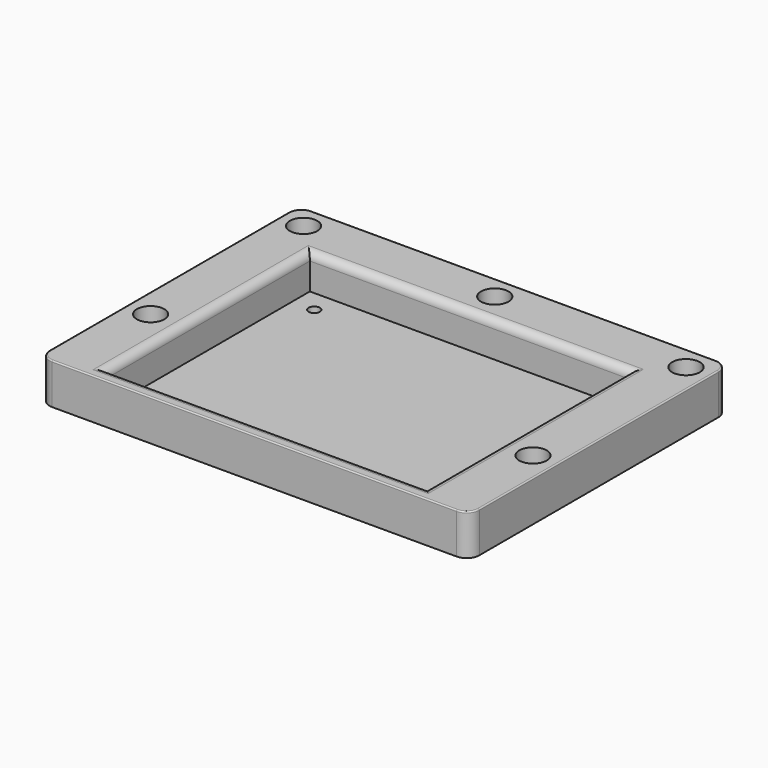
from build123d import *

# Parameters (mm, degrees)
F0_W          = 128.778
F0_H          = 102.108
F1_DEPTH      = 2.54
F2_W          = 173.228
F2_H          = 130.683
F2_W_2        = 128.778
F2_H_2        = 102.108
F3_DEPTH      = 16.51
F4_R          = 3.175
F5_R          = 5.55625
F6_DEPTH      = 16.511
F7_R          = 2.2479
F8_DEPTH      = 2.541
F9_R          = 0.508
F10_T1_DEPTH  = 29.21
F10_T4_ANGLE  = 90
F10_T6_ANGLE  = 90
F10_T8_ANGLE  = 90
F10_T10_ANGLE = 90


# Not quite as in the source:
# - a fillet or chamfer that OpenCascade refuses, or shapes differently, is made with other operations: its cross-section is extruded or revolved along the edge and cut away or added


with BuildPart() as f1:
    # F0 (on Top) → F1 (new body)
    with BuildSketch(Plane.XY):
        Rectangle(F0_W, F0_H)
    extrude(amount=F1_DEPTH)

    # F2 (on Top) → F3 (join)
    with BuildSketch(Plane.XY):
        with Locations((0, 7.9375)):
            Rectangle(F2_W, F2_H)
        Rectangle(F2_W_2, F2_H_2, mode=Mode.SUBTRACT)
    extrude(amount=F3_DEPTH)

    # F4
    f4_edges = [f1.edges().sort_by_distance(p)[0] for p in [
        (-64.389, 0, 16.51),
        (0, 51.054, 16.51),
        (64.389, 0, 16.51),
        (0, -51.054, 16.51),
    ]]
    fillet(f4_edges, radius=F4_R)

    # F5 (on face) → F6 (cut, through all)
    with BuildSketch(Plane.XY.offset(16.51)):
        with Locations((0, 63.754)):
            Circle(F5_R)
        with Locations((77.089, 63.754)):
            Circle(F5_R)
        with Locations((-77.089, 63.754)):
            Circle(F5_R)
        with Locations((-77.089, -13.335)):
            Circle(F5_R)
        with Locations((77.089, -13.335)):
            Circle(F5_R)
    extrude(amount=-F6_DEPTH, mode=Mode.SUBTRACT)

    # F7 (on face) → F8 (cut, through all)
    with BuildSketch(Plane.XY.offset(2.54)):
        with Locations((-55.499, 42.164)):
            Circle(F7_R)
        with Locations((55.499, 42.164)):
            Circle(F7_R)
        with Locations((55.499, -42.164)):
            Circle(F7_R)
        with Locations((-55.499, -42.164)):
            Circle(F7_R)
    extrude(amount=-F8_DEPTH, mode=Mode.SUBTRACT)

    # F9
    f9_edges = [f1.edges().sort_by_distance(p)[0] for p in [
        (0, 73.279, 16.51),
        (-86.614, 7.9375, 16.51),
        (0, -57.404, 16.51),
        (86.614, 7.9375, 16.51),
    ]]
    fillet(f9_edges, radius=F9_R)

    # F10: fillet of radius 5.08 on 4 edges, made by hand

    # F10_s2 → F10_t1 (cut)
    with BuildSketch(Plane.XY.offset(-12.7)):
        with BuildLine():
            ThreePointArc((-81.534, 73.279), (-85.1261024484, 71.7911024484), (-86.614, 68.199))
            Line((-86.614, 68.199), (-86.614, 73.279))
            Line((-86.614, 73.279), (-81.534, 73.279))
        make_face()
        with BuildLine():
            ThreePointArc((-86.614, -52.324), (-85.1261024484, -55.9161024484), (-81.534, -57.404))
            Line((-81.534, -57.404), (-86.614, -57.404))
            Line((-86.614, -57.404), (-86.614, -52.324))
        make_face()
        with BuildLine():
            ThreePointArc((86.614, -52.324), (85.1261024484, -55.9161024484), (81.534, -57.404))
            Line((81.534, -57.404), (86.614, -57.404))
            Line((86.614, -57.404), (86.614, -52.324))
        make_face()
        with BuildLine():
            ThreePointArc((81.534, 73.279), (85.1261024484, 71.7911024484), (86.614, 68.199))
            Line((86.614, 68.199), (86.614, 73.279))
            Line((86.614, 73.279), (81.534, 73.279))
        make_face()
    extrude(amount=F10_T1_DEPTH, mode=Mode.SUBTRACT)

    # F10_s3 → F10_t4 (revolve, cut)
    with BuildSketch(Plane.XZ.offset(-68.199)):
        with BuildLine():
            ThreePointArc((86.106, 16.51), (86.4652102448, 16.3612102448), (86.614, 16.002))
            Line((86.614, 16.002), (86.614, 16.51))
            Line((86.614, 16.51), (86.106, 16.51))
        make_face()
    revolve(axis=Axis((81.534, 68.199, 16.51), (0, 0, 1)), revolution_arc=F10_T4_ANGLE, mode=Mode.SUBTRACT)

    # F10_s5 → F10_t6 (revolve, cut)
    with BuildSketch(Plane.YZ.offset(81.534)):
        with BuildLine():
            ThreePointArc((-56.896, 16.51), (-57.2552102448, 16.3612102448), (-57.404, 16.002))
            Line((-57.404, 16.002), (-57.404, 16.51))
            Line((-57.404, 16.51), (-56.896, 16.51))
        make_face()
    revolve(axis=Axis((81.534, -52.324, 16.51), (0, 0, 1)), revolution_arc=F10_T6_ANGLE, mode=Mode.SUBTRACT)

    # F10_s7 → F10_t8 (revolve, cut)
    with BuildSketch(Plane.XZ.offset(52.324)):
        with BuildLine():
            ThreePointArc((-86.106, 16.51), (-86.4652102448, 16.3612102448), (-86.614, 16.002))
            Line((-86.614, 16.002), (-86.614, 16.51))
            Line((-86.614, 16.51), (-86.106, 16.51))
        make_face()
    revolve(axis=Axis((-81.534, -52.324, 16.51), (0, 0, 1)), revolution_arc=F10_T8_ANGLE, mode=Mode.SUBTRACT)

    # F10_s9 → F10_t10 (revolve, cut)
    with BuildSketch(Plane.YZ.offset(-81.534)):
        with BuildLine():
            ThreePointArc((72.771, 16.51), (73.1302102448, 16.3612102448), (73.279, 16.002))
            Line((73.279, 16.002), (73.279, 16.51))
            Line((73.279, 16.51), (72.771, 16.51))
        make_face()
    revolve(axis=Axis((-81.534, 68.199, 16.51), (0, 0, 1)), revolution_arc=F10_T10_ANGLE, mode=Mode.SUBTRACT)


solid = f1.part
